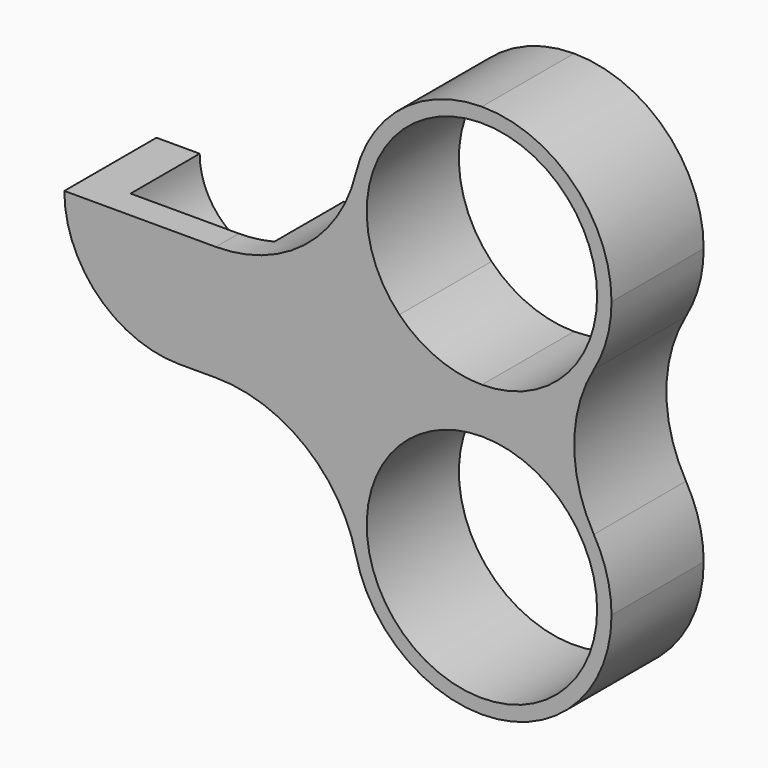
from build123d import *

# Parameters (mm, degrees)
F1_DEPTH = 4
F2_R     = 5
F3_R     = 3.99999
F4_DEPTH = 3


# Not quite as in the source:
# - a fillet or chamfer is up to 0.001 mm smaller than in the source, because OpenCascade refuses the exact size
# - a feature names something its author has since deleted; it is built from what else it names


with BuildPart() as f1:
    # F0 (on Front) → F1 (new body)
    with BuildSketch(Plane.XZ):
        with BuildLine():
            Line((-4.5, -6.79), (-4.5, -2.79))
            Line((-4.5, -2.79), (-8, -2.79))
            ThreePointArc((-8, -2.79), (-10.5, -5.29), (-13, -2.79))
            Line((-13, -2.79), (-14.5, -2.79))
            Line((-14.5, -2.79), (-14.5, -6.79))
            Line((-14.5, -6.79), (-4.5, -6.79))
        make_face()
        with BuildLine():
            ThreePointArc((-13, -2.79), (-10.5, -5.29), (-8, -2.79))
            Line((-8, -2.79), (-13, -2.79))
        make_face()
        with BuildLine():
            Line((-3.5307081443, -2.79), (-4.5, -2.79))
            Line((-4.5, -2.79), (-4.5, -6.79))
            Line((-4.5, -6.79), (-3.5307081443, -6.79))
            ThreePointArc((-3.5307081443, -6.79), (-1.9615045246, -5.53), (0, -5.08))
            Line((0, -5.08), (0, -4.5))
            ThreePointArc((0, -4.5), (-1.9615045246, -4.05), (-3.5307081443, -2.79))
        make_face()
        with BuildLine():
            ThreePointArc((4.5, 0), (3.1819805153, 3.1819805153), (0, 4.5))
            ThreePointArc((0, 4.5), (-3.1819805153, 3.1819805153), (-4.5, 0))
            ThreePointArc((-4.5, 0), (-4.2507756145, -1.4767893131), (-3.5307081443, -2.79))
            Line((-3.5307081443, -2.79), (-2.8663391286, -2.79))
            ThreePointArc((-2.8663391286, -2.79), (-1.5057628442, 3.7057628442), (4, 0))
            ThreePointArc((4, 0), (2.8284271247, -2.8284271247), (0, -4))
            Line((0, -4), (0, -4.5))
            ThreePointArc((0, -4.5), (2.2405062847, -3.9025801194), (3.8861134595, -2.2689473726))
            ThreePointArc((3.8861134595, -2.2689473726), (4.3438180537, -1.1752636794), (4.5, 0))
        make_face()
        with BuildLine():
            Line((-2.8663391286, -2.79), (-3.5307081443, -2.79))
            ThreePointArc((-3.5307081443, -2.79), (-1.9615045246, -4.05), (0, -4.5))
            Line((0, -4.5), (0, -4))
            ThreePointArc((0, -4), (-1.5556349186, -3.6851051545), (-2.8663391286, -2.79))
        make_face()
        with BuildLine():
            ThreePointArc((0, -5.08), (-1.9615045246, -5.53), (-3.5307081443, -6.79))
            Line((-3.5307081443, -6.79), (-2.8663391286, -6.79))
            ThreePointArc((-2.8663391286, -6.79), (-1.5556349186, -5.8948948455), (0, -5.58))
            Line((0, -5.58), (0, -5.08))
        make_face()
        with BuildLine():
            ThreePointArc((4.5, -9.58), (4.3438180596, -8.4047363422), (3.886113482, -7.3110526659))
            ThreePointArc((3.886113482, -7.3110526659), (2.240506304, -5.6774198917), (0, -5.08))
            Line((0, -5.08), (0, -5.58))
            ThreePointArc((0, -5.58), (2.8284271247, -6.7515728753), (4, -9.58))
            ThreePointArc((4, -9.58), (-1.5057628442, -13.2857628442), (-2.8663391286, -6.79))
            Line((-2.8663391286, -6.79), (-3.5307081443, -6.79))
            ThreePointArc((-3.5307081443, -6.79), (-4.2507756145, -8.1032106869), (-4.5, -9.58))
            ThreePointArc((-4.5, -9.58), (-3.1819805153, -12.7619805153), (0, -14.08))
            ThreePointArc((0, -14.08), (3.1819805153, -12.7619805153), (4.5, -9.58))
        make_face()
        with BuildLine():
            Line((-3.5307081443, -6.79), (-4.5, -6.79))
            Line((-4.5, -6.79), (-4.5, -9.58))
            ThreePointArc((-4.5, -9.58), (-4.2507756145, -8.1032106869), (-3.5307081443, -6.79))
        make_face()
        with BuildLine():
            ThreePointArc((-3.5307081443, -2.79), (-4.2507756145, -1.4767893131), (-4.5, 0))
            Line((-4.5, 0), (-4.5, -2.79))
            Line((-4.5, -2.79), (-3.5307081443, -2.79))
        make_face()
        with BuildLine():
            ThreePointArc((3.886113482, -7.3110526659), (3.2040173086, -4.7900000223), (3.8861134595, -2.2689473726))
            ThreePointArc((3.8861134595, -2.2689473726), (2.2405062847, -3.9025801194), (0, -4.5))
            Line((0, -4.5), (0, -5.08))
            ThreePointArc((0, -5.08), (2.240506304, -5.6774198917), (3.886113482, -7.3110526659))
        make_face()
    extrude(amount=F1_DEPTH)

    # F2
    f2_edges = [f1.edges().sort_by_distance(p)[0] for p in [
        (-4.5, -2, -2.79),
        (-4.5, -2, -6.79),
    ]]
    fillet(f2_edges, radius=F2_R)

    # F3 (radius 4 in the source; OpenCascade refuses exactly that, so slightly less here)
    f3_edges = [f1.edges().sort_by_distance(p)[0] for p in [
        (-14.5, -2, -6.79),
    ]]
    fillet(f3_edges, radius=F3_R)

    # F0 (on Front) → F4 (cut)
    with BuildSketch(Plane.XZ):
        with BuildLine():
            ThreePointArc((-13, -2.79), (-10.5, -5.29), (-8, -2.79))
            Line((-8, -2.79), (-13, -2.79))
        make_face()
        with BuildLine():
            Line((-13, -2.79), (-8, -2.79))
            ThreePointArc((-8, -2.79), (-10.5, -0.29), (-13, -2.79))
        make_face()
    extrude(amount=F4_DEPTH, mode=Mode.SUBTRACT)


solid = f1.part
